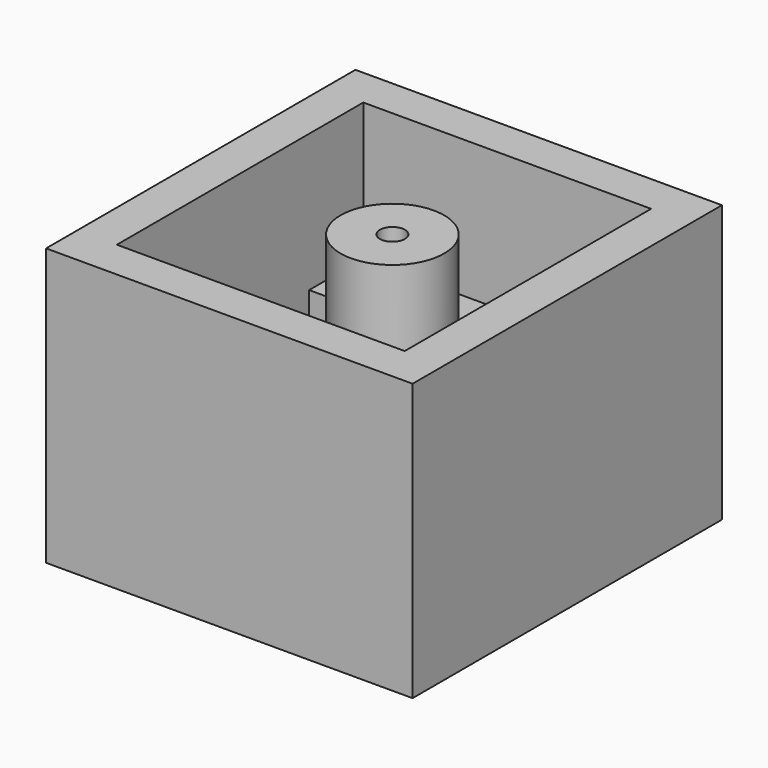
from build123d import *

# Parameters (mm, degrees)
F0_W     = 93.204498291
F0_H     = 98.337136209
F1_DEPTH = 25.4
F2_DEPTH = 45
F4_D     = 6.35
F7_T     = -10
F8_W     = 36.6022491455
F8_H     = 17.213357389
F9_DEPTH = 25.4


# Not quite as in the source:
# - the program builds the solid bodies; features that only make, move or delete a surface that nothing else refers to are left out


with BuildPart() as f1:
    # F0 (on Top) → F1 (new body)
    with BuildSketch(Plane.XY):
        with Locations((-3.3413916826, 1.5083067119)):
            Rectangle(F0_W, F0_H)
    extrude(amount=F1_DEPTH)

    # F2 (add): a face of the model
    f2_faces = [f1.faces().sort_by_distance(p)[0] for p in [
        (-3.3413916826, 1.5083067119, 25.4),
    ]]
    extrude(f2_faces, amount=F2_DEPTH)

    # F4 (through all)
    with Locations(Plane.XY.offset(70.4)):
        with Locations((0, 0)):
            Hole(F4_D / 2)

    # F7
    f7_openings = [f1.faces().sort_by_distance(p)[0] for p in [
        (-3.352977, 1.513536, 70.4),
    ]]
    offset(amount=F7_T, openings=f7_openings)

    # F8 (on face) → F9 (join)
    with BuildSketch(Plane.XY.offset(10)):
        with Locations((-21.6425162554, 32.0701961219)):
            Rectangle(F8_W, F8_H)
    extrude(amount=F9_DEPTH)


solid = f1.part
